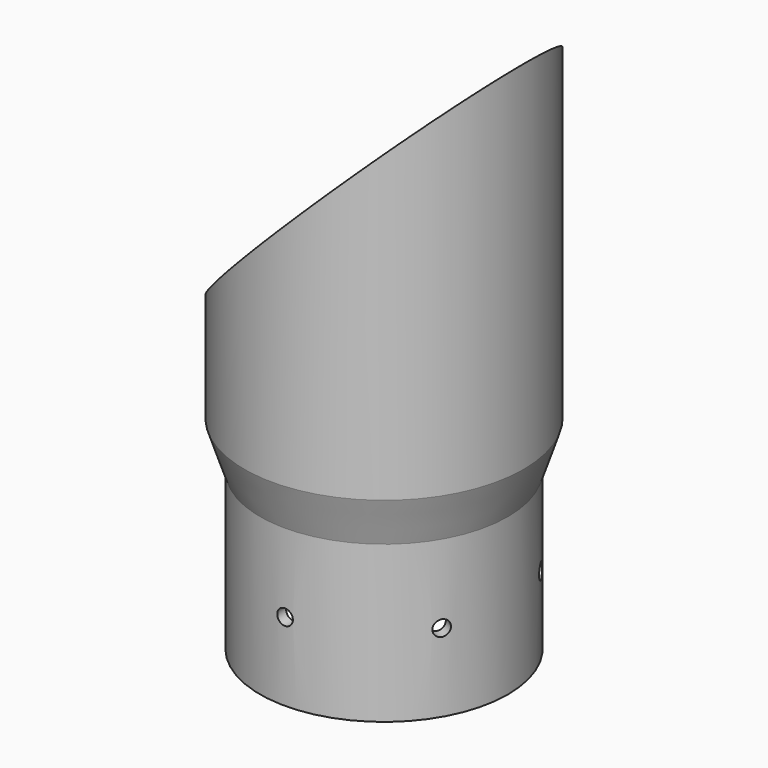
from build123d import *

# Parameters (mm, degrees)
F4_DEPTH        = 50.8
F5_R            = 1.27
F6_DEPTH        = 25.4
F6_COPIES_COUNT = 3
F6_COPIES_ANGLE = 120


# Not quite as in the source:
# - a pattern or mirror of a feature is missing from the dataset's text; its kind, count and spacing are read off the source's solid


with BuildPart() as f2:
    # F0 (on Front) → F2 (revolve)
    with BuildSketch(Plane.XZ):
        Polygon((18.3515, 0), (18.3515, -25.4), (20.1295, -25.4), (20.1295, 0), (22.6695, 7.62), (22.6695, 66.04), (20.8915, 66.04), (20.8915, 7.62), align=None)
    revolve(axis=Axis((0, 0, 6.9738039747), (0, 0, -1)))

    # F3 (on Front) → F4 (cut, symmetric)
    with BuildSketch(Plane.XZ):
        Polygon((-23.876, 146.05), (-23.876, 19.05), (103.124, 146.05), align=None)
    extrude(amount=F4_DEPTH, both=True, mode=Mode.SUBTRACT)

    # F5 (on Front) → F6 (cut, symmetric)
    with BuildSketch(Plane.XZ):
        with Locations((0, -12.7)):
            Circle(F5_R)
    f6 = extrude(amount=F6_DEPTH, both=True, mode=Mode.SUBTRACT)

    # F6_copies: F6 ×3 about axis
    f6_copies_axis = Axis((0, 0, 0), (0, 0, 1))
    for i in range(1, F6_COPIES_COUNT):
        add(f6.rotate(f6_copies_axis, i * F6_COPIES_ANGLE / (F6_COPIES_COUNT - 1)), mode=Mode.SUBTRACT)


solid = f2.part
